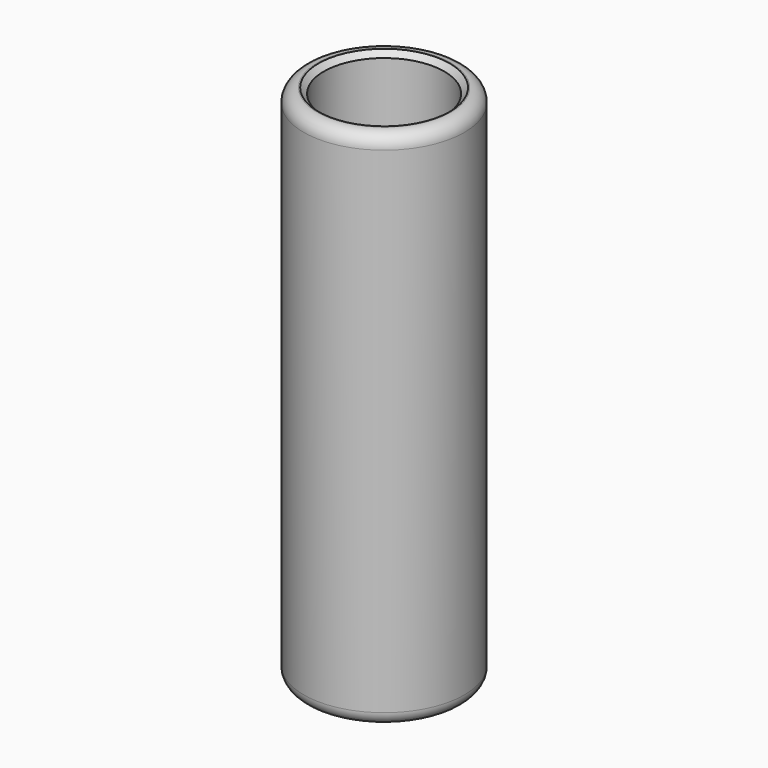
from build123d import *

# Parameters (mm, degrees)
F0_R     = 6
F0_R_2   = 4
F1_DEPTH = 4
F2_DEPTH = 4
F3_R     = 6
F3_R_2   = 4.5
F4_DEPTH = 20
F5_R     = 6
F5_R_2   = 4.45
F6_DEPTH = 15
F7_SIZE  = 0.4
F8_R     = 1


with BuildPart() as f1:
    # F0 (on Top) → F1 (new body)
    with BuildSketch(Plane.XY):
        Circle(F0_R)
        Circle(F0_R_2, mode=Mode.SUBTRACT)
    extrude(amount=F1_DEPTH)

    # F0 (on Top) → F2 (join)
    with BuildSketch(Plane.XY):
        Circle(F0_R)
        Circle(F0_R_2, mode=Mode.SUBTRACT)
    extrude(amount=F2_DEPTH)

    # F3 (on face) → F4 (join)
    with BuildSketch(Plane.XY.offset(4)):
        Circle(F3_R)
        Circle(F3_R_2, mode=Mode.SUBTRACT)
    extrude(amount=F4_DEPTH)

    # F5 (on face) → F6 (join)
    with BuildSketch(Plane(origin=(0, 0, 0), x_dir=(1, 0, 0), z_dir=(0, 0, -1))):
        Circle(F5_R)
        Circle(F5_R_2, mode=Mode.SUBTRACT)
    extrude(amount=F6_DEPTH)

    # F7
    f7_edges = [f1.edges().sort_by_distance(p)[0] for p in [
        (-4.45, 0, -15),
        (-4.5, 0, 24),
    ]]
    chamfer(f7_edges, length=F7_SIZE)

    # F8
    f8_edges = [f1.edges().sort_by_distance(p)[0] for p in [
        (-6, 0, 24),
        (-6, 0, -15),
    ]]
    fillet(f8_edges, radius=F8_R)


solid = f1.part
